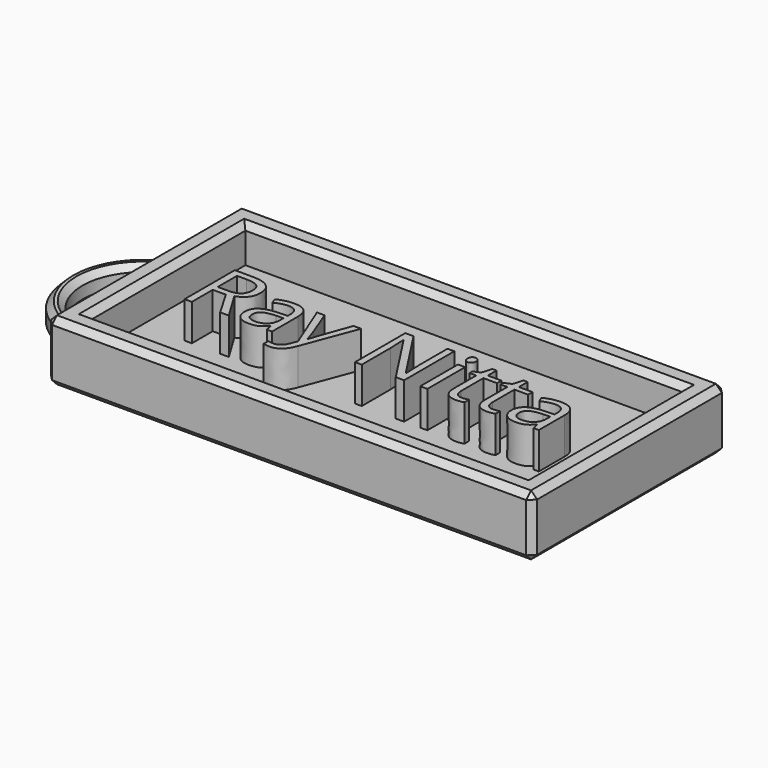
from build123d import *

# Parameters (mm, degrees)
F0_W         = 101.6
F0_H         = 50.8
F1_DEPTH     = 12.7
F2_T         = -5.08
F3_TEXT_SIZE = 18.379020427
F4_DEPTH     = 7.62
F6_DEPTH     = 5.08
F7_SIZE      = 1.27


# Not quite as in the source:
# - Text() gives the source's letters only with a copy of the font that has no kerning and outlines rounded to 1/6400 em; it was checked with that copy


with BuildPart() as f1:
    # F0 (on Top) → F1 (new body)
    with BuildSketch(Plane.XY):
        Rectangle(F0_W, F0_H)
    extrude(amount=F1_DEPTH)

    # F2
    f2_openings = [f1.faces().sort_by_distance(p)[0] for p in [
        (0, 0, 12.7),
    ]]
    offset(amount=F2_T, openings=f2_openings)

    # F3 (on face) → F4 (join, through all)
    with BuildSketch(Plane.XY.offset(5.08)):
        with Locations((-38.6228599673, -6.691722665)):
            Text('Ray Nitta', F3_TEXT_SIZE, font='Open Sans', text_align=(TextAlign.LEFT, TextAlign.BOTTOM))
    extrude(amount=F4_DEPTH)

    # F5 (on Top) → F6 (join)
    with BuildSketch(Plane.XY):
        with BuildLine():
            ThreePointArc((-50.8, 15.875), (-66.675, 0), (-50.8, -15.875))
            Line((-50.8, -15.875), (-50.8, -12.7))
            ThreePointArc((-50.8, -12.7), (-63.5, 0), (-50.8, 12.7))
            Line((-50.8, 12.7), (-50.8, 15.875))
        make_face()
    extrude(amount=F6_DEPTH)

    # F7
    f7_edges = [f1.edges().sort_by_distance(p)[0] for p in [
        (50.8, 0, 12.7),
        (0, 25.4, 12.7),
        (-50.8, 0, 12.7),
        (0, -25.4, 12.7),
        (45.72, 0, 12.7),
        (0, -20.32, 12.7),
        (-45.72, 0, 12.7),
        (0, 20.32, 12.7),
        (50.8, 0, 0),
        (0, 25.4, 0),
        (-50.8, 20.6375, 0),
        (-66.675, 0, 0),
        (-50.8, -20.6375, 0),
        (0, -25.4, 0),
        (-50.8, 0, 0),
        (-63.5, 0, 0),
        (-50.8, 25.4, 6.35),
        (50.8, 25.4, 6.35),
        (50.8, -25.4, 6.35),
        (-50.8, -25.4, 6.35),
        (-66.675, 0, 5.08),
        (-63.5, 0, 5.08),
    ]]
    chamfer(f7_edges, length=F7_SIZE)


solid = f1.part
